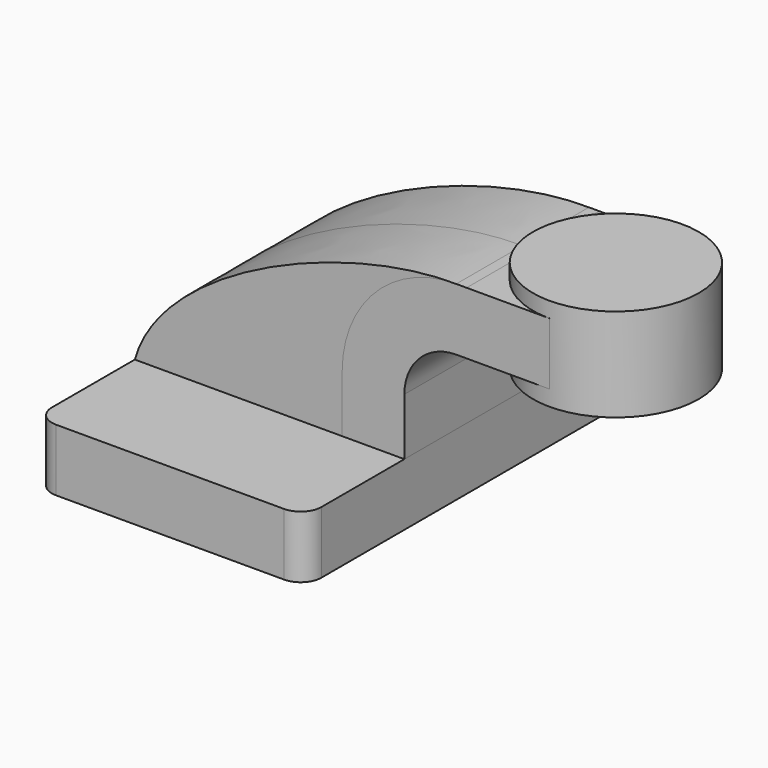
from build123d import *

# Parameters (mm, degrees)
F1_DEPTH = 63.5
F2_DEPTH = 25.4
F3_DEPTH = 25.4
F5_R     = 6.35


# Not quite as in the source:
# - ends of sketch curves that miss each other by under 0.0002 mm in the source are joined
# - a feature names something its author has since deleted; it is built from what else it names


with BuildPart() as f1:
    # F0 (on Front) → F1 (new body, symmetric)
    with BuildSketch(Plane.XZ):
        Polygon((-41.275, 9.525), (-41.275, -9.525), (41.275, -9.525), (41.275, 9.525), (22.2250005586, 9.525), align=None)
    extrude(amount=F1_DEPTH, both=True)

    # F5
    f5_edges = [f1.edges().sort_by_distance(p)[0] for p in [
        (-41.275, -63.5, 0),
        (41.275, -63.5, 0),
        (41.275, 63.5, 0),
        (-41.275, 63.5, 0),
    ]]
    fillet(f5_edges, radius=F5_R)


with BuildPart() as f2:
    # F0 (on Front) → F2 (new body, symmetric)
    with BuildSketch(Plane.XZ):
        with BuildLine():
            Line((22.2250005586, 9.525), (41.275, 9.525))
            Line((41.275, 9.525), (41.275, 27.0002))
            ThreePointArc((41.275, 27.0002), (45.9246798487, 38.2255201513), (57.15, 42.8752))
            Line((57.15, 42.8752), (60.325, 42.8752))
            Line((60.325, 42.8752), (60.325, 61.9251994414))
            Line((60.325, 61.9251994414), (57.15, 61.9251988828))
            ThreePointArc((57.15, 61.9251988828), (32.454296457, 51.695903543), (22.2250011172, 27.0002))
            Line((22.2250011172, 27.0002), (22.2250005586, 9.525))
        make_face()
        Polygon((67.4121566832, 61.9251988828), (60.325, 61.9251988828), (60.325, 42.8752), (85.725, 42.8752), (85.725, 61.9251988828), align=None)
    extrude(amount=F2_DEPTH, both=True)


with BuildPart() as f3:
    # F0 (on Front) → F3 (new body, symmetric)
    with BuildSketch(Plane.XZ):
        with BuildLine():
            add(Edge.make_bspline(
                [(-41.275, 9.525), (-32.9427421093, 39.3494740129), (23.3934521675, 62.3923577368), (57.15, 61.9251988828)],
                knots=[0, 0, 0, 0, 111.5045356385, 111.5045356385, 111.5045356385, 111.5045356385], degree=3))
            Line((-41.275, 9.525), (22.2250005586, 9.525))
            Line((22.2250005586, 9.525), (22.2250011172, 27.0002))
            ThreePointArc((22.2250011172, 27.0002), (32.454296457, 51.695903543), (57.15, 61.9251988828))
        make_face()
    extrude(amount=F3_DEPTH, both=True)


with BuildPart() as f4:
    # F0 (on Front) → F4 (revolve)
    with BuildSketch(Plane.XZ):
        Polygon((85.725, 66.675), (85.725, 61.9251988828), (85.725, 42.8752), (85.725, 38.1), (111.125, 38.1), (111.125, 66.675), align=None)
    revolve(axis=Axis((85.725, 0, 52.4001994414), (0, 0, -1)))


solid = Compound([f1.part, f2.part, f3.part, f4.part])
